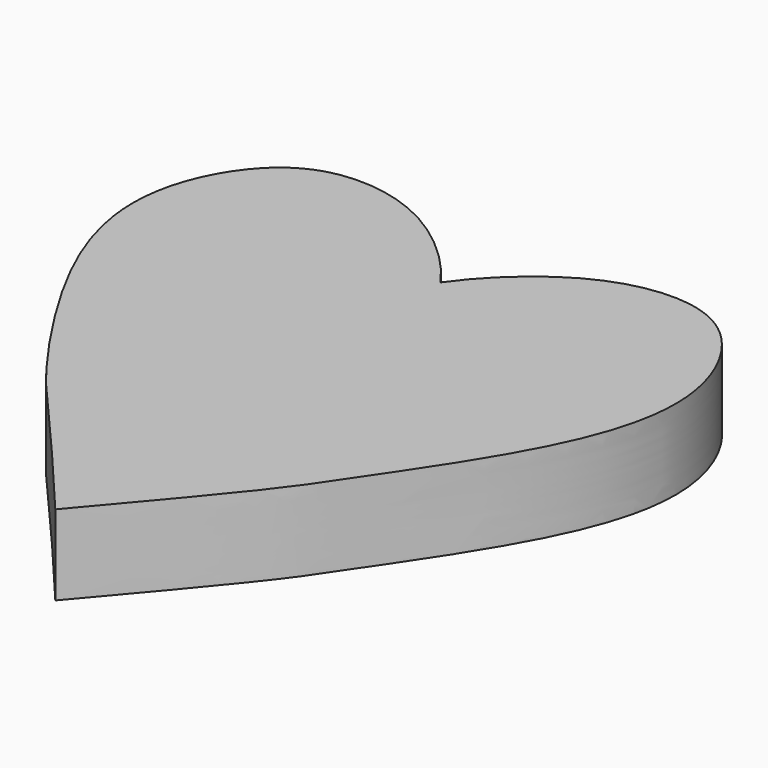
from build123d import *

# Parameters (mm, degrees)
F2_DEPTH = 12.7
F1_R     = 3.9075923968
F1_R_2   = 4.6054442358
F1_R_3   = 3.7178564559
F3_DEPTH = 6.35
F5_DEPTH = 6.2992


# Not quite as in the source:
# - the dataset's text gives a spline's control points without its knots; the knots are read off the source's solid


with BuildPart() as f2:
    # F0 (on Top) → F2 (new body)
    with BuildSketch(Plane.XY):
        with BuildLine():
            add(Edge.make_bspline(
                [(-0.0002192325, 29.7788829798), (1.0311805215, 31.2737992188), (2.9794189406, 33.6632193744), (6.0961829347, 36.7003816582), (8.9218154145, 39.0157025975), (11.8968446345, 41.0287591729), (15.0506182783, 42.6832991355), (17.8386908723, 43.7122624084), (20.1704706167, 44.2949919142), (22.5721025222, 44.7071103266), (25.6637059779, 44.8576351595), (28.7587979148, 44.3963051938), (31.1566280252, 43.580206607), (32.8934233433, 42.72649944), (34.539954123, 41.6112480345), (36.5716871003, 39.8195420038), (38.7986193574, 37.0830062787), (40.5511603087, 33.8617817201), (41.6293314531, 31.0944648379), (42.2648871137, 28.948759753), (42.7154575758, 26.7568386973), (43.0546387967, 23.8092681107), (43.0074663952, 20.0806507913), (42.2579171678, 15.5340260929), (41.1089481353, 11.6757376021), (39.9050000603, 8.5385577207), (38.8672179733, 6.1585608802), (37.6998131399, 3.7466958636), (35.9903190764, 0.4996349429), (33.6383168727, -3.557068685), (30.683709656, -8.2426185492), (28.2903221262, -11.8403909392), (26.5245658284, -14.440576172), (25.3021044485, -16.2275234883), (24.3905435828, -17.5611258944), (23.7409482578, -18.5203243143), (23.1443309204, -19.4095600787), (22.4709834398, -20.4220930943), (21.7064585158, -21.564660073), (20.9136258812, -22.7189057283), (19.7263263678, -24.3808287024), (17.8261099957, -26.8895368015), (14.312326581, -31.2608869978), (8.9860612274, -37.6776773135), (3.8415546052, -43.7738831947), (0.7747457578, -47.3899843653)],
                knots=[0.0141296234, 0.0141296234, 0.0141296234, 0.0141296234, 0.0625, 0.09375, 0.125, 0.15625, 0.1875, 0.21875, 0.234375, 0.25, 0.28125, 0.3125, 0.328125, 0.34375, 0.359375, 0.375, 0.40625, 0.4375, 0.453125, 0.46875, 0.484375, 0.5, 0.53125, 0.5625, 0.59375, 0.609375, 0.625, 0.640625, 0.65625, 0.6875, 0.71875, 0.75, 0.765625, 0.78125, 0.796875, 0.8046875, 0.8125, 0.828125, 0.84375, 0.859375, 0.875, 0.90625, 0.9375, 0.96875, 1, 1, 1, 1], degree=3))
            add(Edge.make_bspline(
                [(-0.0002192325, 29.7788829798), (-1.0331539923, 31.2755086771), (-2.9873225611, 33.6708745587), (-6.1161051719, 36.7177763454), (-8.9523215569, 39.039346061), (-11.9379440654, 41.0545417866), (-15.1027157359, 42.707467346), (-17.9003231377, 43.7320516043), (-20.2401383011, 44.309722088), (-22.6496975377, 44.7154214563), (-25.7498524634, 44.8543528732), (-28.8514635098, 44.3751348271), (-31.252413099, 43.5402923331), (-32.9906367651, 42.6698846484), (-34.6361090953, 41.5367596107), (-36.665684951, 39.7226520697), (-38.8873807242, 36.9593855262), (-40.628214281, 33.7147375481), (-41.6910726777, 30.9315607377), (-42.3117570617, 28.775589446), (-42.7431158553, 26.5755532297), (-43.0523071818, 23.6196189288), (-42.96424568, 19.8819286585), (-42.1699002671, 15.3252141603), (-40.7595222569, 10.6818603695), (-39.1289496736, 6.7248931397), (-37.5816276368, 3.4924198323), (-35.8925628226, 0.2279120246), (-33.5782349973, -3.8485855622), (-30.663218207, -8.5462410284), (-28.2766530793, -12.1382493759), (-26.4869395216, -14.7219183705), (-25.2284680467, -16.4898782692), (-24.0749945536, -18.0667259971), (-23.0579551986, -19.4185170104), (-22.1306432559, -20.6077280272), (-21.2257165865, -21.7220659742), (-20.2824662371, -22.8416465315), (-18.8891886194, -24.4530449727), (-16.7308375611, -26.9035256249), (-12.94422837, -31.2352168827), (-7.4360294024, -37.6452761096), (-2.2690554615, -43.7592729567), (0.7747457578, -47.3899843653)],
                knots=[0.0141243039, 0.0141243039, 0.0141243039, 0.0141243039, 0.0625, 0.09375, 0.125, 0.15625, 0.1875, 0.21875, 0.234375, 0.25, 0.28125, 0.3125, 0.328125, 0.34375, 0.359375, 0.375, 0.40625, 0.4375, 0.453125, 0.46875, 0.484375, 0.5, 0.53125, 0.5625, 0.59375, 0.625, 0.640625, 0.65625, 0.6875, 0.71875, 0.75, 0.765625, 0.78125, 0.796875, 0.8125, 0.828125, 0.84375, 0.859375, 0.875, 0.90625, 0.9375, 0.96875, 1, 1, 1, 1], degree=3))
        make_face()
    extrude(amount=F2_DEPTH)

    # F1 (on face) → F3 (cut)
    with BuildSketch(Plane.XY):
        with BuildLine():
            add(Edge.make_bspline(
                [(0, 21.3432759047), (-5.349304823, 22.1398440835), (-17.0574769564, 44.8808038142), (-36.8386555783, 32.5644167474), (-33.6576402433, 7.3490034133), (-2.6789758311, -31.1789303234), (-0.0952628743, -39.5084778735), (3.4400090716, -31.4657894434), (34.9881125553, 5.749764405), (38.9266017522, 39.4320415347), (11.914565296, 37.2120462512), (4.6062285187, 20.6573596624), (0, 21.3432759047)],
                knots=[0, 0, 0, 0, 0.1086089461, 0.1916939823, 0.2969024381, 0.4503470603, 0.499161772, 0.5476142122, 0.7021170484, 0.8129469407, 0.9064780114, 1, 1, 1, 1], degree=3))
        make_face()
        with Locations((0, -15.9042607993)):
            Circle(F1_R, mode=Mode.SUBTRACT)
        with Locations((-19.0265141428, 20.0266800821)):
            Circle(F1_R_2, mode=Mode.SUBTRACT)
        with Locations((21.9102855772, 18.5805428773)):
            Circle(F1_R_3, mode=Mode.SUBTRACT)
    extrude(amount=F3_DEPTH, mode=Mode.SUBTRACT)

    # F4 (on face) → F5 (cut)
    with BuildSketch(Plane.XY):
        Polygon((27.5262519717, 37.2197963297), (28.9559029043, 44.2712493241), (25.7473737001, 44.7431467474), (24.1323020309, 37.1959805489), align=None)
    extrude(amount=F5_DEPTH, mode=Mode.SUBTRACT)


solid = f2.part
